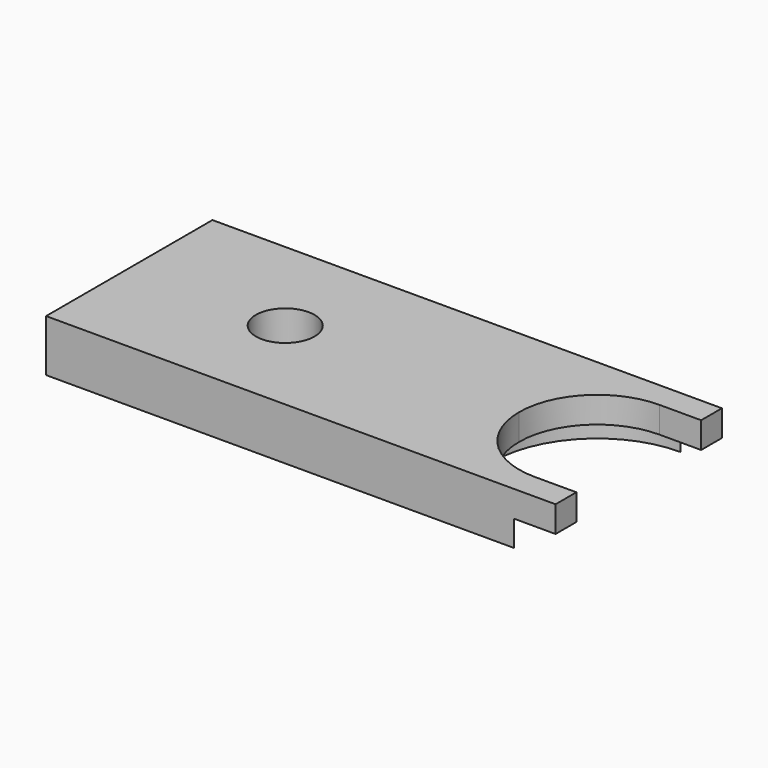
from build123d import *

# Parameters (mm, degrees)
F1_DEPTH = 6.35
F2_W     = 2.54
F2_H     = 9.525
F3_DEPTH = 3.176
F4_W     = 2.54
F4_H     = 1.5875
F4_H_2   = 9.525
F5_DEPTH = 1.5748
F7_D     = 3.5814


with BuildPart() as f1:
    # F0 (on Front) → F1 (new body, symmetric)
    with BuildSketch(Plane.XZ):
        Polygon((0, 3.175), (0, 0), (31.115, 0), (31.115, 1.5875), (31.115, 3.175), align=None)
    extrude(amount=F1_DEPTH, both=True)

    # F2 (on face) → F3 (cut, through all)
    with BuildSketch(Plane.XY.offset(3.175)):
        with BuildLine():
            Line((28.575, -4.7625), (28.575, 4.7625))
            ThreePointArc((28.575, 4.7625), (25.2074039664, 3.3675960572), (23.8125, 3.35e-08))
            ThreePointArc((23.8125, 3.35e-08), (25.2074039428, -3.3675960336), (28.575, -4.7625))
        make_face()
        with Locations((29.845, 0)):
            Rectangle(F2_W, F2_H)
    extrude(amount=-F3_DEPTH, mode=Mode.SUBTRACT)

    # F4 (on face) → F5 (cut)
    with BuildSketch(Plane(origin=(0, 0, 0), x_dir=(1, 0, 0), z_dir=(0, 0, -1))):
        with Locations((29.845, 5.55625)):
            Rectangle(F4_W, F4_H)
        with Locations((29.845, 0)):
            Rectangle(F4_W, F4_H_2)
        with BuildLine():
            Line((28.575, 4.7625), (28.575, 6.35))
            ThreePointArc((28.575, 6.35), (24.0848719273, 4.4901280484), (22.225, -3.44e-08))
            ThreePointArc((22.225, -3.44e-08), (24.0848719516, -4.4901280727), (28.575, -6.35))
            Line((28.575, -6.35), (28.575, -4.7625))
            ThreePointArc((28.575, -4.7625), (23.8125, 0), (28.575, 4.7625))
        make_face()
        Polygon((31.115, -5.55625), (31.115, -4.7625), (28.575, -4.7625), (28.575, -6.35), (31.115, -6.35), align=None)
    extrude(amount=-F5_DEPTH, mode=Mode.SUBTRACT)

    # F7 (through all)
    with Locations(Plane.XY.offset(3.175)):
        with Locations((9.525, 0)):
            Hole(F7_D / 2)


solid = f1.part
